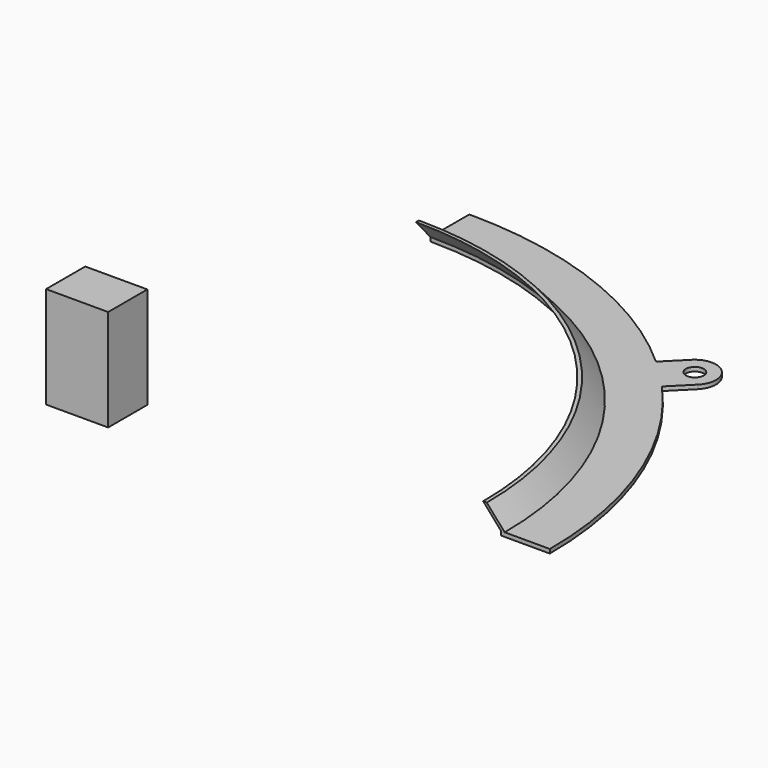
from build123d import *

# Parameters (mm, degrees)
F0_R     = 2.2
F1_DEPTH = 1
F0_W     = 15.2652747326
F0_H     = 12.0394033708
F3_DEPTH = 25
F4_ANGLE = 90


# Not quite as in the source:
# - a feature names something its author has since deleted; it is built from what else it names


with BuildPart() as f1:
    # F0 (on Top) → F1 (new body)
    with BuildSketch(Plane.XY):
        with BuildLine():
            Line((94.5659986717, 82.2709264254), (99.4709712732, 87.1758990269))
            ThreePointArc((99.4709712732, 87.1758990269), (99.4709744308, 94.5298127088), (92.1170607489, 94.5298095512))
            Line((92.1170607489, 94.5298095512), (87.2120881473, 89.6248369497))
            ThreePointArc((87.2120881473, 89.6248369497), (56.4572447999, 108.4651318213), (20.9940191686, 115.0360319122))
            Line((20.9940191686, 115.0360319122), (20.9940191686, 103.0360319122))
            ThreePointArc((20.9940191686, 103.0360319122), (82.5004116823, 77.5592499604), (107.9771936341, 16.0528574467))
            Line((107.9771936341, 16.0528574467), (119.9771936341, 16.0528574467))
            ThreePointArc((119.9771936341, 16.0528574467), (113.4062935433, 51.5160830779), (94.5659986717, 82.2709264254))
        make_face()
        with Locations((95.7940191686, 90.8528574467)):
            Circle(F0_R, mode=Mode.SUBTRACT)
    extrude(amount=F1_DEPTH)

    # F2 (on face) → F4 (revolve)
    with BuildSketch(Plane.XZ.offset(-16.0528574467)):
        Polygon((108.8771936341, 1), (104.4771936341, 6), (103.5771936341, 6), (107.9771936341, 1), align=None)
    revolve(axis=Axis((20.9940191686, 16.0528574467, 12.5), (0, 0, 1)), revolution_arc=F4_ANGLE)


with BuildPart() as f3:
    # F0 (on Top) → F3 (new body)
    with BuildSketch(Plane.XY):
        with Locations((13.3613818023, 10.0331557613)):
            Rectangle(F0_W, F0_H)
    extrude(amount=F3_DEPTH)


solid = Compound([f1.part, f3.part])
